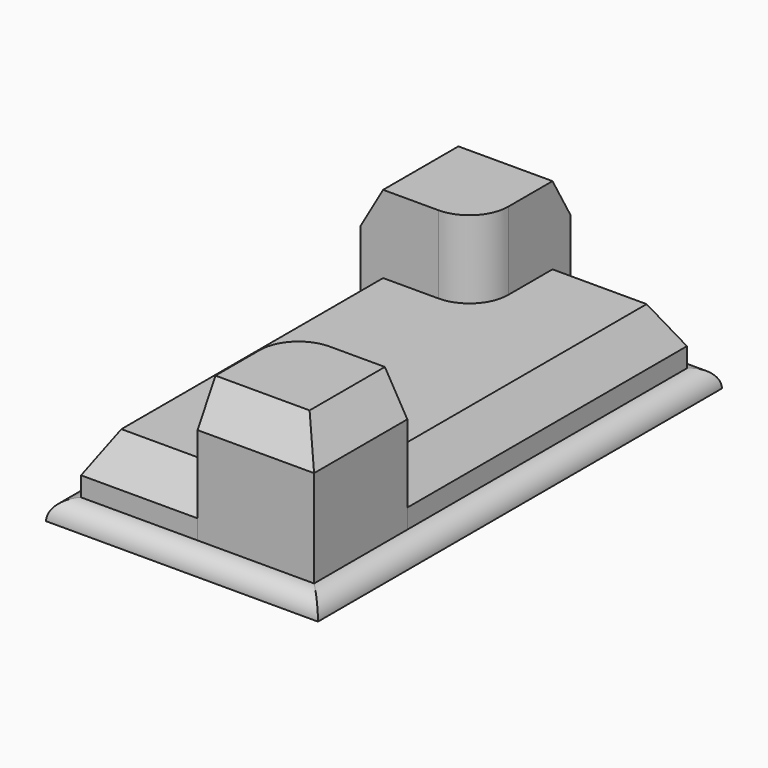
from build123d import *

# Parameters (mm, degrees)
F0_W       = 88.9
F0_H       = 165.1
F1_DEPTH   = 6.35
F2_DEPTH   = 25.4
F3_DEPTH   = 50.8
F4_R       = 6.34999
F5_SIZE2   = 7.3323484187
F5_SIZE    = 12.7
F5_2_SIZE2 = 7.3323484187
F5_2_SIZE  = 12.7
F6_SIZE2   = 7.3323484187
F6_SIZE    = 12.7


# Not quite as in the source:
# - a fillet or chamfer is up to 0.001 mm smaller than in the source, because OpenCascade refuses the exact size


with BuildPart() as f1:
    # F0 (on Top) → F1 (new body)
    with BuildSketch(Plane.XY):
        with Locations((-1.3702638615, -7.1521108847)):
            Rectangle(F0_W, F0_H)
        Polygon((-1.3702638615, -83.3521108847), (-39.4702638615, -83.3521108847), (-39.4702638615, 30.9478891153), (-39.4702638615, 69.0478891153), (-1.3702638615, 69.0478891153), (36.7297361385, 69.0478891153), (36.7297361385, -45.2521108847), (36.7297361385, -83.3521108847), align=None, mode=Mode.SUBTRACT)
    extrude(amount=F1_DEPTH)

    # F4 (radius 6.35 in the source; OpenCascade refuses exactly that, so slightly less here)
    f4_edges = [f1.edges().sort_by_distance(p)[0] for p in [
        (-1.370264, -89.702111, 6.35),
        (43.079736, -7.152111, 6.35),
        (-45.820264, -7.152111, 6.35),
        (-1.370264, 75.397889, 6.35),
    ]]
    fillet(f4_edges, radius=F4_R)


with BuildPart() as f2:
    # F0 (on Top) → F2 (new body)
    with BuildSketch(Plane.XY):
        with BuildLine():
            Line((-39.4702638615, 30.9478891153), (-39.4702638615, -83.3521108847))
            Line((-39.4702638615, -83.3521108847), (-1.3702638615, -83.3521108847))
            Line((-1.3702638615, -83.3521108847), (-1.3702638615, -57.9521108847))
            ThreePointArc((-1.3702638615, -57.9521108847), (2.3494800174, -48.9718547636), (11.3297361385, -45.2521108847))
            Line((11.3297361385, -45.2521108847), (36.7297361385, -45.2521108847))
            Line((36.7297361385, -45.2521108847), (36.7297361385, 69.0478891153))
            Line((36.7297361385, 69.0478891153), (-1.3702638615, 69.0478891153))
            Line((-1.3702638615, 69.0478891153), (-1.3702638615, 43.6478891153))
            ThreePointArc((-1.3702638615, 43.6478891153), (-5.0900077404, 34.6676329943), (-14.0702638615, 30.9478891153))
            Line((-14.0702638615, 30.9478891153), (-39.4702638615, 30.9478891153))
        make_face()
    extrude(amount=F2_DEPTH)

    # F5#2
    f5_2_edges = [f2.edges().sort_by_distance(p)[0] for p in [
        (36.729736, 11.897889, 25.4),
        (17.679736, 69.047889, 25.4),
        (-39.470264, -26.202111, 25.4),
        (-20.420264, -83.352111, 25.4),
    ]]
    chamfer(f5_2_edges, length=F5_2_SIZE, length2=F5_2_SIZE2)


with BuildPart() as f3:
    # F0 (on Top) → F3 (new body)
    with BuildSketch(Plane.XY):
        with BuildLine():
            Line((-39.4702638615, 69.0478891153), (-39.4702638615, 30.9478891153))
            Line((-39.4702638615, 30.9478891153), (-14.0702638615, 30.9478891153))
            ThreePointArc((-14.0702638615, 30.9478891153), (-5.0900077404, 34.6676329943), (-1.3702638615, 43.6478891153))
            Line((-1.3702638615, 43.6478891153), (-1.3702638615, 69.0478891153))
            Line((-1.3702638615, 69.0478891153), (-39.4702638615, 69.0478891153))
        make_face()
    extrude(amount=F3_DEPTH)

    # F6
    f6_edges = [f3.edges().sort_by_distance(p)[0] for p in [
        (-20.420264, 69.047889, 50.8),
        (-39.470264, 49.997889, 50.8),
    ]]
    chamfer(f6_edges, length=F6_SIZE, length2=F6_SIZE2)


with BuildPart() as f3b:
    # F0 (on Top) → F3, piece 2 (new body)
    with BuildSketch(Plane.XY):
        with BuildLine():
            Line((-1.3702638615, -57.9521108847), (-1.3702638615, -83.3521108847))
            Line((-1.3702638615, -83.3521108847), (36.7297361385, -83.3521108847))
            Line((36.7297361385, -83.3521108847), (36.7297361385, -45.2521108847))
            Line((36.7297361385, -45.2521108847), (11.3297361385, -45.2521108847))
            ThreePointArc((11.3297361385, -45.2521108847), (2.3494800174, -48.9718547636), (-1.3702638615, -57.9521108847))
        make_face()
    extrude(amount=F3_DEPTH)

    # F5
    f5_edges = [f3b.edges().sort_by_distance(p)[0] for p in [
        (17.679736, -83.352111, 50.8),
        (36.729736, -64.302111, 50.8),
    ]]
    chamfer(f5_edges, length=F5_SIZE, length2=F5_SIZE2)


solid = Compound([f1.part, f2.part, f3.part, f3b.part])
